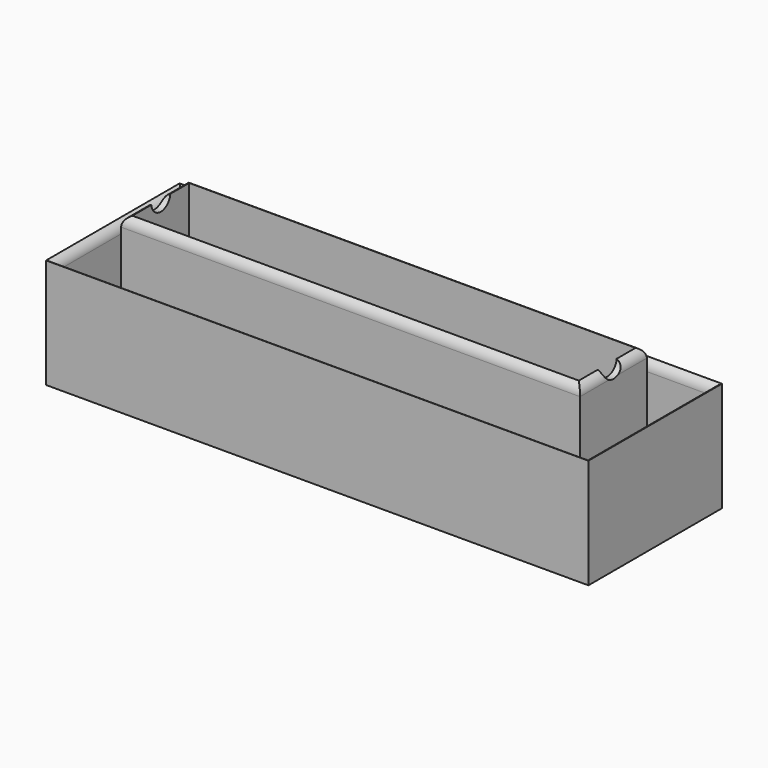
from build123d import *

# Parameters (mm, degrees)
F0_W          = 260
F0_H          = 80
F1_DEPTH      = 1
F2_W          = 10
F2_H          = 10
F3_DEPTH      = 50
F4_T          = 1
F4_T3_DEPTH   = 12
F4_T5_DEPTH   = 12
F4_T7_DEPTH   = 12
F4_T9_DEPTH   = 12
F5_W          = 260
F5_H          = 80
F6_DEPTH      = 3
F7_W          = 260
F7_H          = 80
F7_W_2        = 254
F7_H_2        = 74
F8_DEPTH      = 50
F9_W          = 220
F9_H          = 40
F10_DEPTH     = 67
F11_W         = 214
F11_H         = 34
F12_DEPTH     = 52
F13_W         = 214
F13_H         = 34
F14_DEPTH     = 15
F15_T1_DEPTH  = 245
F15_T3_DEPTH  = 65
F15_T5_DEPTH  = 254
F15_T7_DEPTH  = 74
F15_T13_DEPTH = 86.5
F15_T19_DEPTH = 266.5
F15_T28_DEPTH = 86.5
F15_T34_DEPTH = 266.5
F15_T43_DEPTH = 266.5
F15_T49_DEPTH = 86.5
F15_T58_DEPTH = 86.5
F15_T64_DEPTH = 266.5
F16_R         = 5.7285158572
F17_DEPTH     = 500
F18_W         = 260
F18_H         = 80
F19_DEPTH     = 51


# Not quite as in the source:
# - a fillet or chamfer that OpenCascade refuses, or shapes differently, is made with other operations: its cross-section is extruded or revolved along the edge and cut away or added
# - a shell that OpenCascade refuses in one call is made with other operations: the cavity is built on its own and cut out


with BuildPart() as f1:
    # F0 (on Top) → F1 (new body)
    with BuildSketch(Plane.XY):
        Rectangle(F0_W, F0_H)
    extrude(amount=F1_DEPTH)

    # F2 (on face) → F3 (join)
    with BuildSketch(Plane.XY.offset(1)):
        with Locations((-125, 35)):
            Rectangle(F2_W, F2_H)
        with Locations((125, 35)):
            Rectangle(F2_W, F2_H)
        with Locations((-125, -35)):
            Rectangle(F2_W, F2_H)
        with Locations((125, -35)):
            Rectangle(F2_W, F2_H)
    extrude(amount=F3_DEPTH)

    # F4: shell of thickness 1, made by hand


with BuildPart() as f4_core1:
    # F4_t2: copy of F1
    add(f1.part)

    # the walls: a layer under each face that stays
    f4_faces = [f4_core1.faces().sort_by_distance(p)[0] for p in [
        (121.3333333333, 40, 49.3),
        (-121.3333333333, -40, 49.3),
        (125, -35, 51),
        (125, -30, 26),
        (120, -35, 26),
        (-120, -35, 26),
        (-125, -30, 26),
        (-125, -35, 51),
        (-130, 34.2857142857, 47.3571428571),
        (-125, 30, 26),
        (-125, 35, 51),
        (-120, 35, 26),
        (0, 0, 1),
        (125, 30, 26),
        (120, 35, 26),
        (125, 35, 51),
        (130, -34.2857142857, 47.3571428571),
    ]]
    thicken(f4_faces, amount=-F4_T, mode=Mode.SUBTRACT)

    # F4_s4 → F4_t3 (cut)
    with BuildSketch(Plane.YZ.offset(119)):
        Polygon((-29.99, 1.01), (-31, 1), (-31, 0), (-30, 0), align=None)
        Polygon((29.99, 1.01), (30, 0), (31, 0), (31, 1), align=None)
    extrude(amount=F4_T3_DEPTH, mode=Mode.SUBTRACT)

    # F4_s6 → F4_t5 (cut)
    with BuildSketch(Plane.XZ.offset(29)):
        Polygon((119.99, 1.01), (121, 1), (121, 0), (120, 0), align=None)
        Polygon((-119.99, 1.01), (-121, 1), (-121, 0), (-120, 0), align=None)
    extrude(amount=F4_T5_DEPTH, mode=Mode.SUBTRACT)

    # F4_s8 → F4_t7 (cut)
    with BuildSketch(Plane.YZ.offset(-131)):
        Polygon((-29.99, 1.01), (-31, 1), (-31, 0), (-30, 0), align=None)
        Polygon((29.99, 1.01), (31, 1), (31, 0), (30, 0), align=None)
    extrude(amount=F4_T7_DEPTH, mode=Mode.SUBTRACT)

    # F4_s10 → F4_t9 (cut)
    with BuildSketch(Plane.XZ.offset(-41)):
        Polygon((-119.99, 1.01), (-121, 1), (-121, 0), (-120, 0), align=None)
        Polygon((119.99, 1.01), (120, 0), (121, 0), (121, 1), align=None)
    extrude(amount=F4_T9_DEPTH, mode=Mode.SUBTRACT)


with BuildPart() as f1_1:
    add(f1.part)

    # what is left inside the walls is the cavity
    f4_cavity = [f4_core1.part.solids().sort_by_distance(p)[0] for p in [
        (125, 38.99, 33.333333),
        (-125, 38.99, 33.333333),
        (128.99, -35, 33.333333),
        (-123.666667, -31.01, 25),
    ]]
    add(f4_cavity, mode=Mode.SUBTRACT)

    # F5 (on face) → F6 (join)
    with BuildSketch(Plane.XY.offset(51)):
        Rectangle(F5_W, F5_H)
    extrude(amount=F6_DEPTH)

    # F7 (on face) → F8 (join)
    with BuildSketch(Plane.XY.offset(54)):
        Rectangle(F7_W, F7_H)
        Rectangle(F7_W_2, F7_H_2, mode=Mode.SUBTRACT)
    extrude(amount=F8_DEPTH)

    # F9 (on face) → F10 (join)
    with BuildSketch(Plane.XY.offset(54)):
        Rectangle(F9_W, F9_H)
    extrude(amount=F10_DEPTH)

    # F11 (on face) → F12 (cut)
    with BuildSketch(Plane.XY.offset(121)):
        Rectangle(F11_W, F11_H)
    extrude(amount=-F12_DEPTH, mode=Mode.SUBTRACT)

    # F13 (on face) → F14 (cut)
    with BuildSketch(Plane(origin=(0, 0, 51), x_dir=(1, 0, 0), z_dir=(0, 0, -1))):
        Rectangle(F13_W, F13_H)
    extrude(amount=-F14_DEPTH, mode=Mode.SUBTRACT)

    # F15: fillet of radius 5 on 8 edges, made by hand

    # F15_s2 → F15_t1 (cut)
    with BuildSketch(Plane.YZ.offset(-122.5)):
        with BuildLine():
            ThreePointArc((-20, 116), (-18.5355339059, 119.5355339059), (-15, 121))
            Line((-15, 121), (-20, 121))
            Line((-20, 121), (-20, 116))
        make_face()
        with BuildLine():
            ThreePointArc((20, 116), (18.5355339059, 119.5355339059), (15, 121))
            Line((15, 121), (20, 121))
            Line((20, 121), (20, 116))
        make_face()
    extrude(amount=F15_T1_DEPTH, mode=Mode.SUBTRACT)

    # F15_s4 → F15_t3 (cut)
    with BuildSketch(Plane.XZ.offset(-32.5)):
        with BuildLine():
            ThreePointArc((-110, 116), (-108.5355339059, 119.5355339059), (-105, 121))
            Line((-105, 121), (-110, 121))
            Line((-110, 121), (-110, 116))
        make_face()
        with BuildLine():
            ThreePointArc((110, 116), (108.5355339059, 119.5355339059), (105, 121))
            Line((105, 121), (110, 121))
            Line((110, 121), (110, 116))
        make_face()
    extrude(amount=F15_T3_DEPTH, mode=Mode.SUBTRACT)

    # F15_s6 → F15_t5 (cut)
    with BuildSketch(Plane.YZ.offset(-127)):
        with BuildLine():
            ThreePointArc((-42, 104), (-38.4644660941, 102.5355339059), (-37, 99))
            Line((-37, 99), (-37, 104))
            Line((-37, 104), (-42, 104))
        make_face()
        with BuildLine():
            ThreePointArc((42, 104), (38.4644660941, 102.5355339059), (37, 99))
            Line((37, 99), (37, 104))
            Line((37, 104), (42, 104))
        make_face()
    extrude(amount=F15_T5_DEPTH, mode=Mode.SUBTRACT)

    # F15_s8 → F15_t7 (cut)
    with BuildSketch(Plane.XZ.offset(-37)):
        with BuildLine():
            ThreePointArc((132, 104), (128.4644660941, 102.5355339059), (127, 99))
            Line((127, 99), (127, 104))
            Line((127, 104), (132, 104))
        make_face()
        with BuildLine():
            ThreePointArc((-132, 104), (-128.4644660941, 102.5355339059), (-127, 99))
            Line((-127, 99), (-127, 104))
            Line((-127, 104), (-132, 104))
        make_face()
    extrude(amount=F15_T7_DEPTH, mode=Mode.SUBTRACT)


with BuildPart() as f15_tool11:
    # F15_s12 → F15_t13 (new body)
    with BuildSketch(Plane.XZ.offset(-37)):
        with BuildLine():
            ThreePointArc((132, 104), (128.4644660941, 102.5355339059), (127, 99))
            Line((127, 99), (127, 104))
            Line((127, 104), (132, 104))
        make_face()
    extrude(amount=F15_T13_DEPTH)

    split(bisect_by=Plane.YZ.offset(130), keep=Keep.BOTTOM)

    split(bisect_by=Plane.XZ.offset(40), keep=Keep.BOTTOM)

    split(bisect_by=Plane.XZ.offset(37), keep=Keep.TOP)


with BuildPart() as f15_tool17:
    # F15_s18 → F15_t19 (new body)
    with BuildSketch(Plane.YZ.offset(139.5)):
        with BuildLine():
            ThreePointArc((-42, 104), (-38.4644660941, 102.5355339059), (-37, 99))
            Line((-37, 99), (-37, 104))
            Line((-37, 104), (-42, 104))
        make_face()
    extrude(amount=-F15_T19_DEPTH)

    split(bisect_by=Plane.YZ.offset(130), keep=Keep.BOTTOM)

    split(bisect_by=Plane.XZ.offset(40), keep=Keep.BOTTOM)

    split(bisect_by=Plane.YZ.offset(127), keep=Keep.TOP)


with BuildPart() as f15_tool11_1:
    add(f15_tool11.part)

    # F15_t23: intersect F15_tool17
    add(f15_tool17.part, mode=Mode.INTERSECT)


with BuildPart() as f1_2:
    add(f1_1.part)

    # F15_t9: cut F15_tool11
    add(f15_tool11_1.part, mode=Mode.SUBTRACT)


with BuildPart() as f15_tool26:
    # F15_s27 → F15_t28 (new body)
    with BuildSketch(Plane.XZ.offset(49.5)):
        with BuildLine():
            ThreePointArc((-132, 104), (-128.4644660941, 102.5355339059), (-127, 99))
            Line((-127, 99), (-127, 104))
            Line((-127, 104), (-132, 104))
        make_face()
    extrude(amount=-F15_T28_DEPTH)

    split(bisect_by=Plane.YZ.offset(-130), keep=Keep.TOP)

    split(bisect_by=Plane.XZ.offset(40), keep=Keep.BOTTOM)

    split(bisect_by=Plane.XZ.offset(37), keep=Keep.TOP)


with BuildPart() as f15_tool32:
    # F15_s33 → F15_t34 (new body)
    with BuildSketch(Plane.YZ.offset(127)):
        with BuildLine():
            ThreePointArc((-42, 104), (-38.4644660941, 102.5355339059), (-37, 99))
            Line((-37, 99), (-37, 104))
            Line((-37, 104), (-42, 104))
        make_face()
    extrude(amount=-F15_T34_DEPTH)

    split(bisect_by=Plane.YZ.offset(-130), keep=Keep.TOP)

    split(bisect_by=Plane.XZ.offset(40), keep=Keep.BOTTOM)

    split(bisect_by=Plane.YZ.offset(-127), keep=Keep.BOTTOM)


with BuildPart() as f15_tool26_1:
    add(f15_tool26.part)

    # F15_t38: intersect F15_tool32
    add(f15_tool32.part, mode=Mode.INTERSECT)


with BuildPart() as f1_3:
    add(f1_2.part)

    # F15_t24: cut F15_tool26
    add(f15_tool26_1.part, mode=Mode.SUBTRACT)


with BuildPart() as f15_tool41:
    # F15_s42 → F15_t43 (new body)
    with BuildSketch(Plane.YZ.offset(-127)):
        with BuildLine():
            ThreePointArc((42, 104), (38.4644660941, 102.5355339059), (37, 99))
            Line((37, 99), (37, 104))
            Line((37, 104), (42, 104))
        make_face()
    extrude(amount=F15_T43_DEPTH)

    split(bisect_by=Plane.XZ.offset(-40), keep=Keep.TOP)

    split(bisect_by=Plane.YZ.offset(130), keep=Keep.BOTTOM)

    split(bisect_by=Plane.YZ.offset(127), keep=Keep.TOP)


with BuildPart() as f15_tool47:
    # F15_s48 → F15_t49 (new body)
    with BuildSketch(Plane.XZ.offset(-49.5)):
        with BuildLine():
            ThreePointArc((132, 104), (128.4644660941, 102.5355339059), (127, 99))
            Line((127, 99), (127, 104))
            Line((127, 104), (132, 104))
        make_face()
    extrude(amount=F15_T49_DEPTH)

    split(bisect_by=Plane.XZ.offset(-40), keep=Keep.TOP)

    split(bisect_by=Plane.YZ.offset(130), keep=Keep.BOTTOM)

    split(bisect_by=Plane.XZ.offset(-37), keep=Keep.BOTTOM)


with BuildPart() as f15_tool41_1:
    add(f15_tool41.part)

    # F15_t53: intersect F15_tool47
    add(f15_tool47.part, mode=Mode.INTERSECT)


with BuildPart() as f1_4:
    add(f1_3.part)

    # F15_t39: cut F15_tool41
    add(f15_tool41_1.part, mode=Mode.SUBTRACT)


with BuildPart() as f15_tool56:
    # F15_s57 → F15_t58 (new body)
    with BuildSketch(Plane.XZ.offset(37)):
        with BuildLine():
            ThreePointArc((-132, 104), (-128.4644660941, 102.5355339059), (-127, 99))
            Line((-127, 99), (-127, 104))
            Line((-127, 104), (-132, 104))
        make_face()
    extrude(amount=-F15_T58_DEPTH)

    split(bisect_by=Plane.XZ.offset(-40), keep=Keep.TOP)

    split(bisect_by=Plane.YZ.offset(-130), keep=Keep.TOP)

    split(bisect_by=Plane.XZ.offset(-37), keep=Keep.BOTTOM)


with BuildPart() as f15_tool62:
    # F15_s63 → F15_t64 (new body)
    with BuildSketch(Plane.YZ.offset(-139.5)):
        with BuildLine():
            ThreePointArc((42, 104), (38.4644660941, 102.5355339059), (37, 99))
            Line((37, 99), (37, 104))
            Line((37, 104), (42, 104))
        make_face()
    extrude(amount=F15_T64_DEPTH)

    split(bisect_by=Plane.XZ.offset(-40), keep=Keep.TOP)

    split(bisect_by=Plane.YZ.offset(-130), keep=Keep.TOP)

    split(bisect_by=Plane.YZ.offset(-127), keep=Keep.BOTTOM)


with BuildPart() as f15_tool56_1:
    add(f15_tool56.part)

    # F15_t68: intersect F15_tool62
    add(f15_tool62.part, mode=Mode.INTERSECT)


with BuildPart() as f1_5:
    add(f1_4.part)

    # F15_t54: cut F15_tool56
    add(f15_tool56_1.part, mode=Mode.SUBTRACT)

    # F16 (on face) → F17 (cut)
    with BuildSketch(Plane.YZ.offset(110)):
        with Locations((0, 121.0692673922)):
            Circle(F16_R)
    extrude(amount=-F17_DEPTH, mode=Mode.SUBTRACT)

    # F18 (on face) → F19 (cut)
    with BuildSketch(Plane(origin=(0, 0, 0), x_dir=(1, 0, 0), z_dir=(0, 0, -1))):
        Rectangle(F18_W, F18_H)
    extrude(amount=-F19_DEPTH, mode=Mode.SUBTRACT)


solid = f1_5.part
